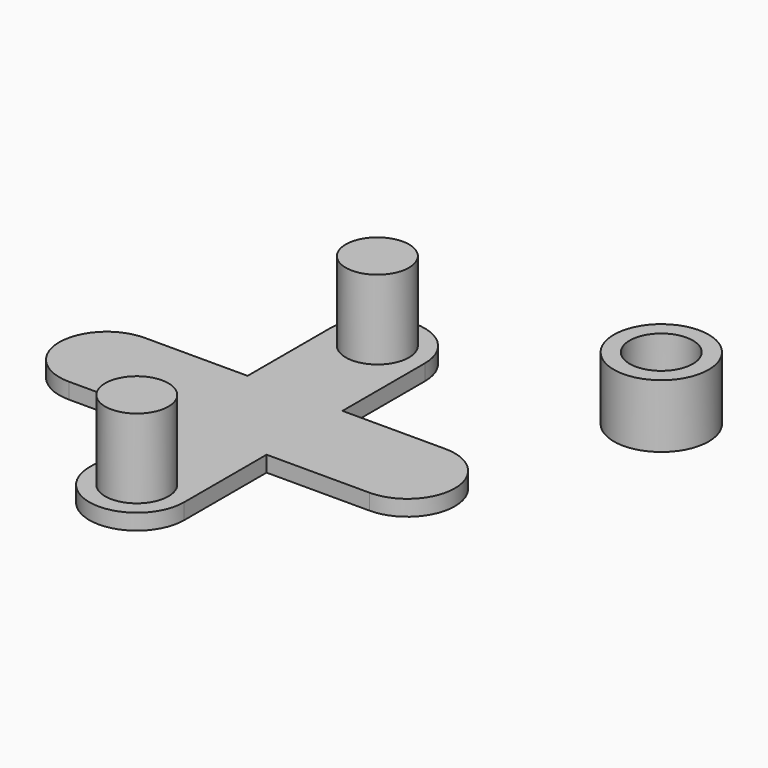
from build123d import *

# Parameters (mm, degrees)
F0_W     = 7.5
F0_H     = 15
F1_DEPTH = 2.5
F2_R     = 5
F3_DEPTH = 12.5
F4_R     = 7.5
F4_R_2   = 5
F5_DEPTH = 10


# Not quite as in the source:
# - a feature names something its author has since deleted; it is built from what else it names


with BuildPart() as f1:
    # F0 (on Top) → F1 (new body)
    with BuildSketch(Plane.XY):
        with BuildLine():
            Line((0, -16.2764129074), (0, -7.5))
            Line((0, -7.5), (-7.5, -7.5))
            Line((-7.5, -7.5), (-7.5, -23.7764129074))
            ThreePointArc((-7.5, -23.7764129074), (-5.3033008589, -18.4731120485), (0, -16.2764129074))
        make_face()
        with Locations((-3.75, 0)):
            Rectangle(F0_W, F0_H)
        with BuildLine():
            Line((0, 7.5), (0, 16.2764129074))
            ThreePointArc((0, 16.2764129074), (-5.3033008589, 18.4731120485), (-7.5, 23.7764129074))
            Line((-7.5, 23.7764129074), (-7.5, 7.5))
            Line((-7.5, 7.5), (0, 7.5))
        make_face()
        with BuildLine():
            ThreePointArc((2.3176274578, 16.6434890352), (1.1732584878, 16.3687503529), (0, 16.2764129074))
            Line((0, 16.2764129074), (0, 7.5))
            Line((0, 7.5), (5.2885271376, 7.5))
            Line((5.2885271376, 7.5), (2.3176274578, 16.6434890352))
        make_face()
        with BuildLine():
            Line((7.5, -7.5), (5.2885271376, -7.5))
            Line((5.2885271376, -7.5), (2.3176274578, -16.6434890352))
            ThreePointArc((2.3176274578, -16.6434890352), (6.0676274578, -19.3680235152), (7.5, -23.7764129074))
            Line((7.5, -23.7764129074), (7.5, -7.5))
        make_face()
        with BuildLine():
            Line((0, -23.7764129074), (0, -16.2764129074))
            ThreePointArc((0, -16.2764129074), (-5.3033008589, -18.4731120485), (-7.5, -23.7764129074))
            ThreePointArc((-7.5, -23.7764129074), (0, -31.2764129074), (7.5, -23.7764129074))
            ThreePointArc((7.5, -23.7764129074), (6.0676274578, -19.3680235152), (2.3176274578, -16.6434890352))
            Line((2.3176274578, -16.6434890352), (0, -23.7764129074))
        make_face()
        with BuildLine():
            ThreePointArc((2.3176274578, -16.6434890352), (1.1732584878, -16.3687503529), (0, -16.2764129074))
            Line((0, -16.2764129074), (0, -23.7764129074))
            Line((0, -23.7764129074), (2.3176274578, -16.6434890352))
        make_face()
        with BuildLine():
            ThreePointArc((7.5, 23.7764129074), (6.0676274578, 19.3680235152), (2.3176274578, 16.6434890352))
            Line((2.3176274578, 16.6434890352), (5.2885271376, 7.5))
            Line((5.2885271376, 7.5), (7.5, 7.5))
            Line((7.5, 7.5), (7.5, 23.7764129074))
        make_face()
        with BuildLine():
            Line((0, 16.2764129074), (0, 23.7764129074))
            Line((0, 23.7764129074), (2.3176274578, 16.6434890352))
            ThreePointArc((2.3176274578, 16.6434890352), (6.0676274578, 19.3680235152), (7.5, 23.7764129074))
            ThreePointArc((7.5, 23.7764129074), (0, 31.2764129074), (-7.5, 23.7764129074))
            ThreePointArc((-7.5, 23.7764129074), (-5.3033008589, 18.4731120485), (0, 16.2764129074))
        make_face()
        with BuildLine():
            Line((2.3176274578, 16.6434890352), (0, 23.7764129074))
            Line((0, 23.7764129074), (0, 16.2764129074))
            ThreePointArc((0, 16.2764129074), (1.1732584878, 16.3687503529), (2.3176274578, 16.6434890352))
        make_face()
        with BuildLine():
            Line((5.2885271376, -7.5), (0, -7.5))
            Line((0, -7.5), (0, -16.2764129074))
            ThreePointArc((0, -16.2764129074), (1.1732584878, -16.3687503529), (2.3176274578, -16.6434890352))
            Line((2.3176274578, -16.6434890352), (5.2885271376, -7.5))
        make_face()
        Polygon((7.5, -0.6937863786), (5.2885271376, -7.5), (7.5, -7.5), align=None)
        Polygon((7.5, 7.5), (5.2885271376, 7.5), (7.5, 0.6937863786), align=None)
        with BuildLine():
            Line((23.7764129074, 7.5), (7.5, 7.5))
            Line((7.5, 7.5), (7.5, 0.6937863786))
            Line((7.5, 0.6937863786), (7.7254248594, 0))
            Line((7.7254248594, 0), (7.5, -0.6937863786))
            Line((7.5, -0.6937863786), (7.5, -7.5))
            Line((7.5, -7.5), (23.7764129074, -7.5))
            ThreePointArc((23.7764129074, -7.5), (16.2764129074, 0), (23.7764129074, 7.5))
        make_face()
        Polygon((5.2885271376, 7.5), (0, 7.5), (0, -7.5), (5.2885271376, -7.5), (7.5, -0.6937863786), (7.5, 0.6937863786), align=None)
        Polygon((7.7254248594, 0), (7.5, 0.6937863786), (7.5, -0.6937863786), align=None)
        with BuildLine():
            ThreePointArc((31.2764129074, 0), (29.0797137663, 5.3033008589), (23.7764129074, 7.5))
            ThreePointArc((23.7764129074, 7.5), (16.2764129074, 0), (23.7764129074, -7.5))
            ThreePointArc((23.7764129074, -7.5), (29.0797137663, -5.3033008589), (31.2764129074, 0))
        make_face()
        with BuildLine():
            Line((-7.5, -7.5), (-7.5, 7.5))
            Line((-7.5, 7.5), (-23.7764129074, 7.5))
            ThreePointArc((-23.7764129074, 7.5), (-18.4731120485, 5.3033008589), (-16.2764129074, 0))
            ThreePointArc((-16.2764129074, 0), (-18.4731120485, -5.3033008589), (-23.7764129074, -7.5))
            Line((-23.7764129074, -7.5), (-7.5, -7.5))
        make_face()
        with BuildLine():
            ThreePointArc((-16.2764129074, 0), (-18.4731120485, 5.3033008589), (-23.7764129074, 7.5))
            ThreePointArc((-23.7764129074, 7.5), (-31.2764129074, 0), (-23.7764129074, -7.5))
            ThreePointArc((-23.7764129074, -7.5), (-18.4731120485, -5.3033008589), (-16.2764129074, 0))
        make_face()
    extrude(amount=F1_DEPTH)

    # F2 (on face) → F3 (join)
    with BuildSketch(Plane.XY.offset(2.5)):
        with Locations((0, 23.7764129074)):
            Circle(F2_R)
        with Locations((0, -23.7764129074)):
            Circle(F2_R)
    extrude(amount=F3_DEPTH)


with BuildPart() as f5:
    # F4 (on Top) → F5 (new body)
    with BuildSketch(Plane.XY):
        with Locations((37.4355688691, 33.1056714058)):
            Circle(F4_R)
        with Locations((37.4355688691, 33.1056714058)):
            Circle(F4_R_2, mode=Mode.SUBTRACT)
    extrude(amount=F5_DEPTH)


solid = Compound([f1.part, f5.part])
